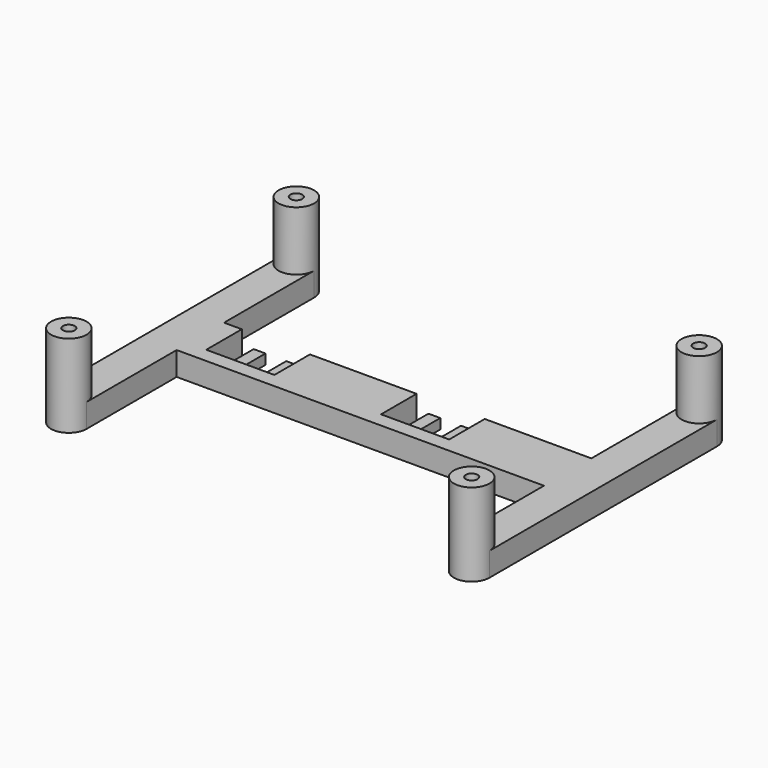
from build123d import *

# Parameters (mm, degrees)
F1_DEPTH = 4
F2_W     = 2
F2_H     = 7.5
F3_DEPTH = 1.7
F5_DEPTH = 10
F6_R     = 1
F7_DEPTH = 25


with BuildPart() as f1:
    # F0 (on Top) → F1 (new body)
    with BuildSketch(Plane.XY):
        with BuildLine():
            Line((6, 0), (68, 0))
            Line((68, 0), (68, -19))
            ThreePointArc((68, -19), (71, -22), (74, -19))
            Line((74, -19), (74, 29))
            ThreePointArc((74, 29), (71, 32), (68, 29))
            Line((68, 29), (68, 10))
            Line((68, 10), (50, 10))
            Line((50, 10), (50, 2.5))
            Line((50, 2.5), (38.5, 2.5))
            Line((38.5, 2.5), (38.5, 10))
            Line((38.5, 10), (20.5, 10))
            Line((20.5, 10), (20.5, 2.5))
            Line((20.5, 2.5), (9, 2.5))
            Line((9, 2.5), (9, 10))
            Line((9, 10), (6, 10))
            Line((6, 10), (6, 29))
            ThreePointArc((6, 29), (3, 32), (0, 29))
            Line((0, 29), (0, -19))
            ThreePointArc((0, -19), (3, -22), (6, -19))
            Line((6, -19), (6, 0))
        make_face()
    extrude(amount=F1_DEPTH)

    # F2 (on Top) → F3 (join)
    with BuildSketch(Plane.XY):
        with Locations((12, 6.25)):
            Rectangle(F2_W, F2_H)
        with Locations((17.5, 6.25)):
            Rectangle(F2_W, F2_H)
        with Locations((41.5, 6.25)):
            Rectangle(F2_W, F2_H)
        with Locations((47, 6.25)):
            Rectangle(F2_W, F2_H)
    extrude(amount=F3_DEPTH)

    # F4 (on face) → F5 (join)
    with BuildSketch(Plane.XY.offset(4)):
        with BuildLine():
            ThreePointArc((0, 29), (3, 26), (6, 29))
            ThreePointArc((6, 29), (3, 32), (0, 29))
        make_face()
        with BuildLine():
            ThreePointArc((6, -19), (3, -16), (0, -19))
            ThreePointArc((0, -19), (3, -22), (6, -19))
        make_face()
        with BuildLine():
            ThreePointArc((74, -19), (71, -16), (68, -19))
            ThreePointArc((68, -19), (71, -22), (74, -19))
        make_face()
        with BuildLine():
            ThreePointArc((68, 29), (71, 26), (74, 29))
            ThreePointArc((74, 29), (71, 32), (68, 29))
        make_face()
    extrude(amount=F5_DEPTH)

    # F6 (on face) → F7 (cut)
    with BuildSketch(Plane(origin=(0, 0, 0), x_dir=(1, 0, 0), z_dir=(0, 0, -1))):
        with Locations((3, 19)):
            Circle(F6_R)
        with Locations((71, 19)):
            Circle(F6_R)
        with Locations((71, -29)):
            Circle(F6_R)
        with Locations((3, -29)):
            Circle(F6_R)
    extrude(amount=-F7_DEPTH, mode=Mode.SUBTRACT)


solid = f1.part
